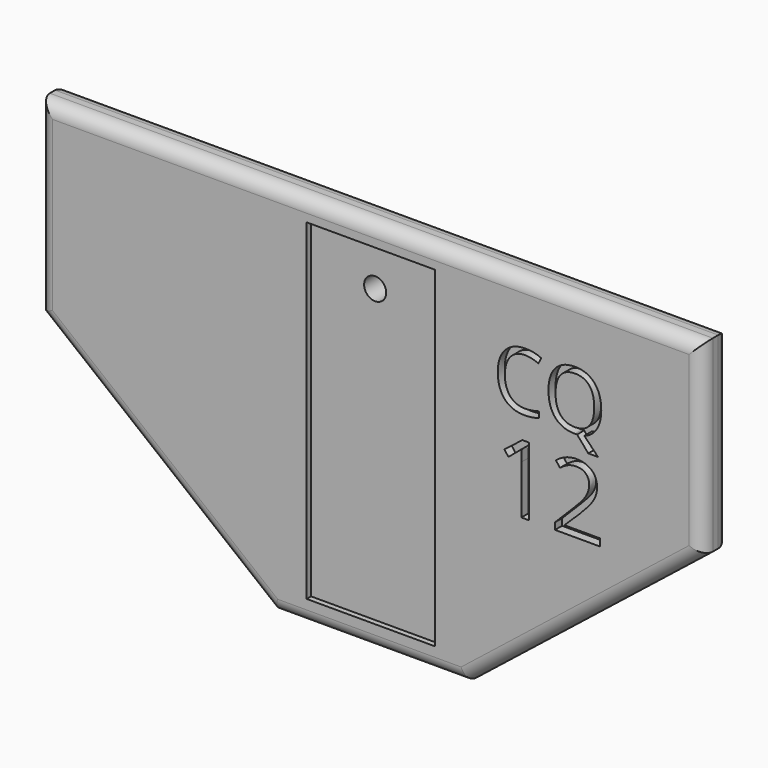
from build123d import *

# Parameters (mm, degrees)
F0_R           = 6.35
F1_DEPTH       = 19.05
F2_W           = 73.66
F2_H           = 190.5
F2_R           = 6.35
F3_DEPTH       = 3.175
F4_R           = 7.62
F5_TEXT_SIZE   = 55.0826959726
F5_TEXT_SIZE_2 = 46.1847185054
F6_DEPTH       = 5.08
F7_R           = 9.8603661503
F8_DEPTH       = 2.54


# Not quite as in the source:
# - Text() gives the source's letters only with a copy of the font that has no kerning and outlines rounded to 1/6400 em; it was checked with that copy


with BuildPart() as f1:
    # F0 (on Front) → F1 (new body)
    with BuildSketch(Plane.XZ):
        Polygon((190.5, 169.0208791231), (-190.5, 169.0208791231), (-190.5, 61.0708791231), (-56.1334975064, -46.8791208769), (54.6081326902, -46.8791208769), (190.5, 61.0708791231), align=None)
        with Locations((0, 133.8931848888)):
            Circle(F0_R, mode=Mode.SUBTRACT)
    extrude(amount=F1_DEPTH)

    # F2 (on face) → F3 (cut)
    with BuildSketch(Plane.XZ.offset(19.05)):
        with Locations((0, 61.5585812122)):
            Rectangle(F2_W, F2_H)
        with Locations((0, 133.8931848888)):
            Circle(F2_R, mode=Mode.SUBTRACT)
    extrude(amount=-F3_DEPTH, mode=Mode.SUBTRACT)

    # F4
    f4_edges = [f1.edges().sort_by_distance(p)[0] for p in [
        (0, -19.05, 169.020879),
        (190.5, -19.05, 115.045879),
        (-0.762682, -19.05, -46.879121),
        (-190.5, -19.05, 115.045879),
        (0, 0, 169.020879),
        (-190.5, 0, 115.045879),
        (-0.762682, 0, -46.879121),
        (190.5, 0, 115.045879),
        (-123.316749, -19.05, 7.095879),
        (122.554066, -19.05, 7.095879),
        (-123.316749, 0, 7.095879),
        (122.554066, 0, 7.095879),
    ]]
    fillet(f4_edges, radius=F4_R)

    # F5 (on face) → F6 (cut)
    with BuildSketch(Plane.XZ.offset(19.05)):
        with Locations((71.6922357678, 47.6307310164)):
            Text('12', F5_TEXT_SIZE, font='Open Sans', text_align=(TextAlign.LEFT, TextAlign.BOTTOM))
        with Locations((70.1668746769, 100.4084367305)):
            Text('CQ', F5_TEXT_SIZE_2, font='Open Sans', text_align=(TextAlign.LEFT, TextAlign.BOTTOM))
    extrude(amount=-F6_DEPTH, mode=Mode.SUBTRACT)

    # F7 (on face) → F8 (cut)
    with BuildSketch(Plane(origin=(0, 0, 0), x_dir=(-1, 0, 0), z_dir=(0, 1, 0))):
        with Locations((0, 133.8931848888)):
            Circle(F7_R)
    extrude(amount=-F8_DEPTH, mode=Mode.SUBTRACT)


solid = f1.part
